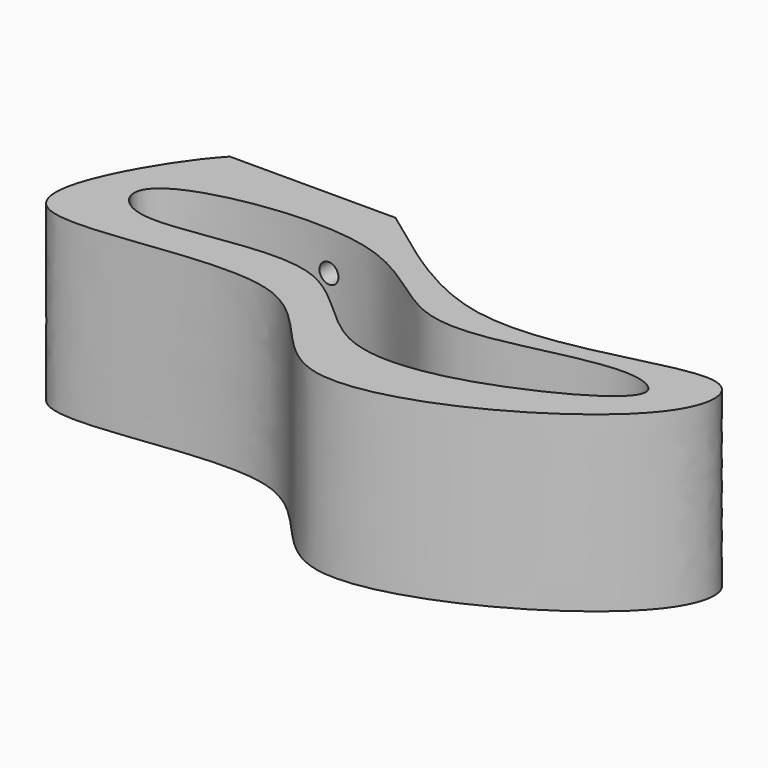
from build123d import *

# Parameters (mm, degrees)
F1_DEPTH = 44.45
F2_W     = 74.2719661038
F2_H     = 19.1847047539
F3_DEPTH = 44.45
F4_R     = 2.54
F5_DEPTH = 12.7
F7_DEPTH = 44.45


with BuildPart() as f1:
    # F0 (on Top) → F1 (new body)
    with BuildSketch(Plane.XY):
        with BuildLine():
            add(Edge.make_bspline(
                [(-48.6255437136, 41.4480604231), (-40.8484346021, 55.0020290598), (-14.5381640102, 84.9118531153), (36.7872341853, 15.3518841758), (103.6097074974, 50.9717063324), (105.366018034, 18.8456481989), (26.2552876949, -24.1944861357), (13.0044728222, 29.9237755732), (-64.2692054709, 3.2811392732), (-54.7940018694, 30.6976534039), (-48.6255437136, 41.4480604231)],
                knots=[0, 0, 0, 0, 0.1201130587, 0.2743919181, 0.4159551531, 0.4889533194, 0.6490342071, 0.7634236695, 0.9047316469, 1, 1, 1, 1], degree=3))
        make_face()
    extrude(amount=F1_DEPTH)

    # F2 (on face) → F3 (cut)
    with BuildSketch(Plane.XY.offset(44.45)):
        with Locations((-0.8888949474, 65.780006769)):
            Rectangle(F2_W, F2_H)
    extrude(amount=-F3_DEPTH, mode=Mode.SUBTRACT)

    # F4 (on face) → F5 (cut)
    with BuildSketch(Plane(origin=(0, 56.187654392, 0), x_dir=(-1, 0, 0), z_dir=(0, 1, 0))):
        with Locations((28.4216627479, 8.9450003579)):
            Circle(F4_R)
        with Locations((28.4216627479, 34.3450003579)):
            Circle(F4_R)
        with Locations((3.0216627479, 8.9450003579)):
            Circle(F4_R)
        with Locations((3.0216627479, 34.3450003579)):
            Circle(F4_R)
    extrude(amount=-F5_DEPTH, mode=Mode.SUBTRACT)

    # F6 (on face) → F7 (cut, through all)
    with BuildSketch(Plane.XY.offset(44.45)):
        with BuildLine():
            add(Edge.make_bspline(
                [(-37.3570807278, 38.5467633605), (-41.6358987226, 36.3675978685), (-45.3251278471, 31.2438646318), (-34.6849049278, 20.9447558378), (8.7684742603, 36.2216119824), (27.8337360027, 1.3076300709), (68.6021829277, 10.8943057633), (95.9868479622, 27.6786171098), (82.6566932331, 35.0590130187), (55.7931561454, 27.179696289), (32.1805583139, 24.8310097681), (11.2256838696, 49.0120466754), (-27.8388621677, 43.3943108507), (-37.3570807278, 38.5467633605)],
                knots=[0, 0, 0, 0, 0.0557984382, 0.1130612418, 0.2291726734, 0.3326582888, 0.4480454993, 0.540551477, 0.5918656122, 0.6898008412, 0.776364443, 0.8758765316, 1, 1, 1, 1], degree=3))
        make_face()
    extrude(amount=-F7_DEPTH, mode=Mode.SUBTRACT)


solid = f1.part
